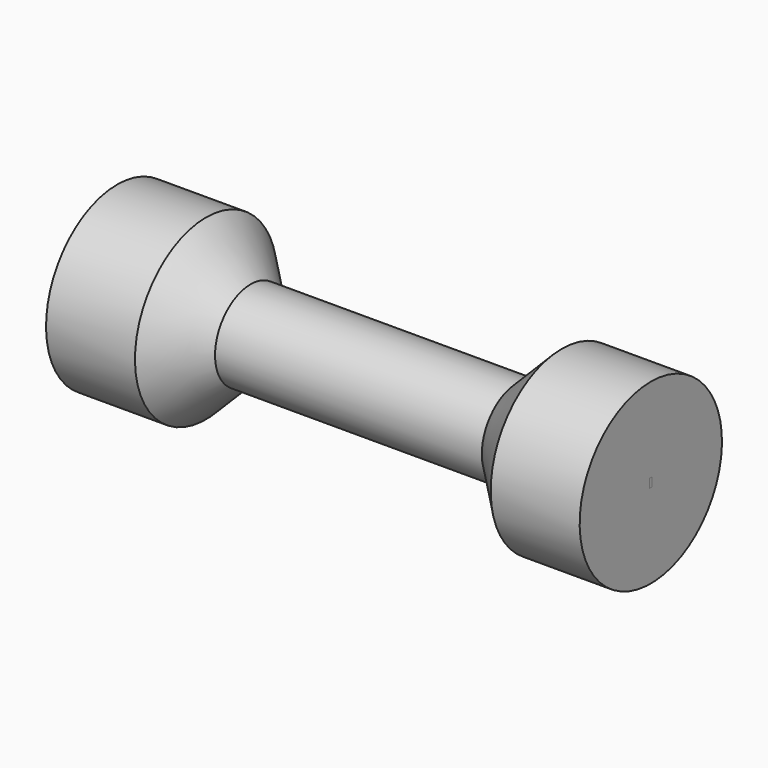
from build123d import *

# Parameters (mm, degrees)
F3_W = 0.2
F3_H = 0.5


with BuildPart() as f1:
    # F0 (on Front) → F1 (revolve)
    with BuildSketch(Plane.XZ):
        Polygon((0, 5), (0, 0), (30, 0), (30, 5), (25, 5), (22.5, 2.5), (7.5, 2.5), (5, 5), align=None)
    revolve(axis=Axis((15, 0, 0), (1, 0, 0)))

    # F5: sweep along a path in F2
    with BuildLine(Plane.XZ) as f5_path:
        Line((0, 0), (30, 0))
    # F3 (on face) → F5 (sweep, cut)
    with BuildSketch(Plane.YZ.offset(30)):
        Rectangle(F3_W, F3_H)
    sweep(path=f5_path.line, mode=Mode.SUBTRACT)


with BuildPart() as f4:
    # F4: sweep along a path in F2
    with BuildLine(Plane.XZ) as f4_path:
        Line((0, 0), (30, 0))
    # F3 (on face) → F4 (sweep)
    with BuildSketch(Plane.YZ.offset(30)):
        Rectangle(F3_W, F3_H)
    sweep(path=f4_path.line)


solid = Compound([f1.part, f4.part])
